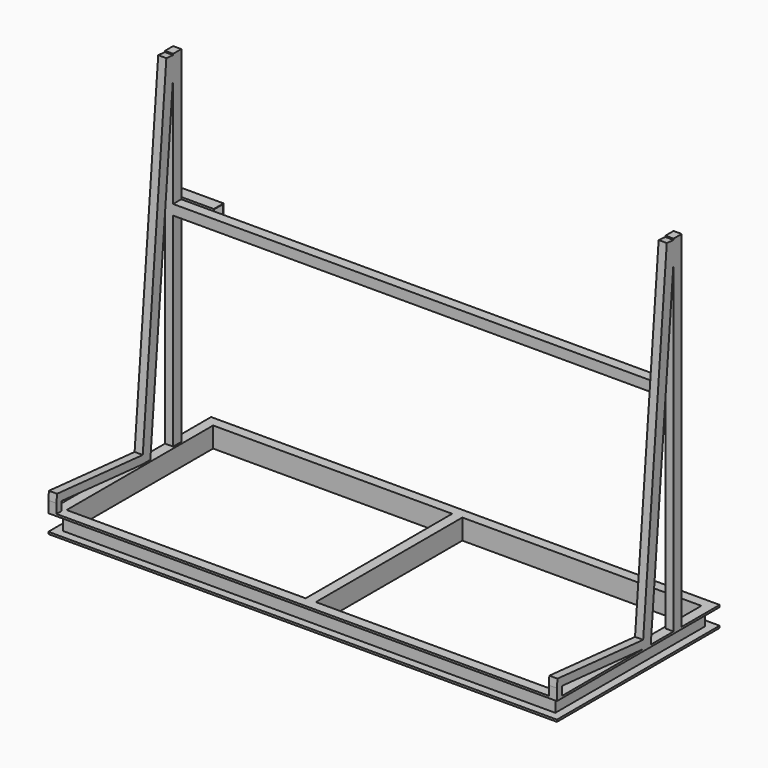
from build123d import *

# Parameters (mm, degrees)
F0_W          = 2500
F0_H          = 1000
F0_W_2        = 1175
F0_H_2        = 900
F1_DEPTH      = 100
F2_W          = 40
F2_H          = 80
F3_DEPTH      = 2500.001
F4_W          = 40
F4_H          = 80
F5_DEPTH      = 960.001
F6_W          = 90
F6_H          = 80
F7_DEPTH      = 450
F7_DEPTH_BACK = 450
F9_DEPTH      = 40
F11_W         = 50
F11_H         = 50
F12_DEPTH     = 2420
F13_W         = 60
F13_H         = 60
F13_W_2       = 55
F13_H_2       = 55
F14_DEPTH     = 200


# Not quite as in the source:
# - a feature names something its author has since deleted; it is built from what else it names


with BuildPart() as f1:
    # F0 (on Top) → F1 (new body)
    with BuildSketch(Plane.XY):
        Rectangle(F0_W, F0_H)
        with Locations((-612.5, 0)):
            Rectangle(F0_W_2, F0_H_2, mode=Mode.SUBTRACT)
        with Locations((612.5, 0)):
            Rectangle(F0_W_2, F0_H_2, mode=Mode.SUBTRACT)
    extrude(amount=F1_DEPTH)

    # F2 (on face) → F3 (cut, through all)
    with BuildSketch(Plane(origin=(-1250, 0, 0), x_dir=(0, -1, 0), z_dir=(-1, 0, 0))):
        with Locations((-480, 50)):
            Rectangle(F2_W, F2_H)
        with Locations((480, 50)):
            Rectangle(F2_W, F2_H)
    extrude(amount=-F3_DEPTH, mode=Mode.SUBTRACT)

    # F4 (on face) → F5 (cut, through all)
    with BuildSketch(Plane.XZ.offset(460)):
        with Locations((1230, 50)):
            Rectangle(F4_W, F4_H)
        with Locations((-1230, 50)):
            Rectangle(F4_W, F4_H)
    extrude(amount=-F5_DEPTH, mode=Mode.SUBTRACT)

    # F6 (on Front) → F7 (cut, two sides)
    with BuildSketch(Plane.XZ) as f7_sk:
        with Locations((-45, 50)):
            Rectangle(F6_W, F6_H)
    extrude(amount=-F7_DEPTH, mode=Mode.SUBTRACT)
    extrude(f7_sk.sketch, amount=F7_DEPTH_BACK, mode=Mode.SUBTRACT)

    # F8 (on face) → F9 (join)
    with BuildSketch(Plane(origin=(-1250, 0, 0), x_dir=(0, -1, 0), z_dir=(-1, 0, 0))):
        Polygon((-216.7047621673, 1700.2073223866), (-76.7047621673, 100), (-26.5137702901, 100), (-30, 139.8477879237), (-175.0597899337, 1797.8887738934), (-216.7047621673, 1794.2453109301), align=None)
        Polygon((-224.8695248383, 1793.530986756), (-216.7047621673, 1700.2073223866), (-216.7047621673, 1794.2453109301), align=None)
        Polygon((-30, 139.8477879237), (-26.5137702901, 100), (468.9004319267, 143.3431264437), (500, 146.0639860907), (500.0249770351, 146.0661712981), (496.5387473252, 185.9139592218), align=None)
        Polygon((500, 146.0639860907), (468.9004319267, 143.3431264437), (468.9004319267, 100), (500, 100), align=None)
        Polygon((-216.7047621673, 100), (-216.7047621673, 1700.2073223866), (-224.8695248383, 1793.530986756), (-216.7047621673, 1794.2453109301), (-216.7047621673, 1800), (-266.7047621673, 1800), (-266.7047621673, 100), align=None)
    extrude(amount=-F9_DEPTH)

    # F10: F1 across plane


with BuildPart() as f1_1:
    add(f1.part)
    add(f1.part.mirror(Plane.YZ))

    # F11 (on face) → F12 (join, through all)
    with BuildSketch(Plane.YZ.offset(-1210)):
        with Locations((241.7047621673, 1125)):
            Rectangle(F11_W, F11_H)
    extrude(amount=F12_DEPTH)

    # F13 (on face) → F14 (join)
    with BuildSketch(Plane(origin=(-1250, 0, 0), x_dir=(0, -1, 0), z_dir=(-1, 0, 0))):
        with Locations((-296.7047621673, 1130)):
            Rectangle(F13_W, F13_H)
        with Locations((-296.7047621673, 1130)):
            Rectangle(F13_W_2, F13_H_2, mode=Mode.SUBTRACT)
    extrude(amount=-F14_DEPTH)


solid = f1_1.part
